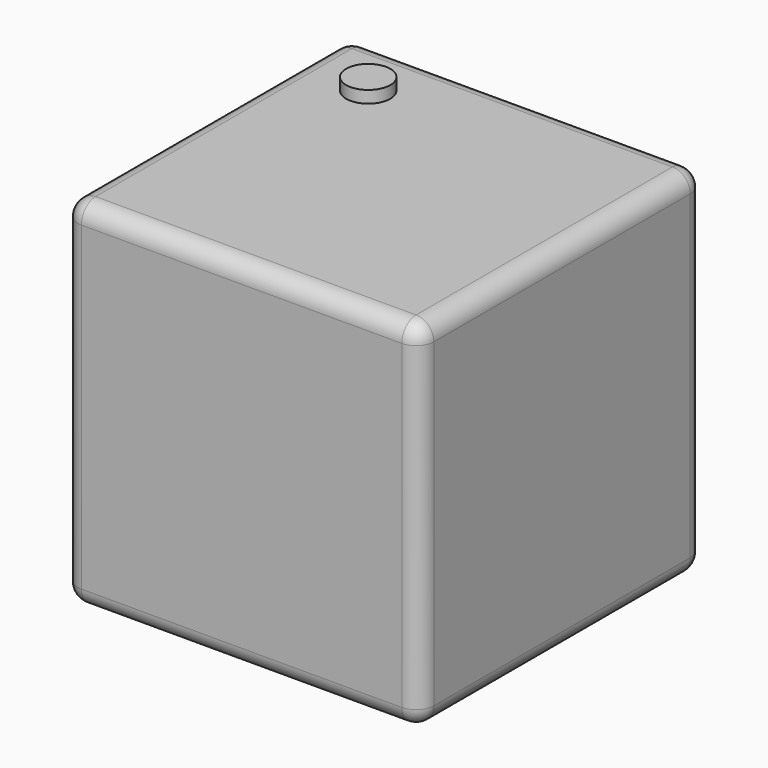
from build123d import *

# Parameters (mm, degrees)
F0_W         = 100
F0_H         = 100
F1_DEPTH     = 100
F2_R         = 5
F3_W         = 84.485553205
F3_H         = 83.5751444101
F4_DEPTH     = 96.9
F5_R         = 5
F6_T1_DEPTH  = 84.485553205
F6_T3_DEPTH  = 83.5751444101
F6_T9_DEPTH  = 96.985553205
F6_T13_DEPTH = 96.0751444101
F6_T20_DEPTH = 96.985553205
F6_T24_DEPTH = 96.0751444101
F6_T31_DEPTH = 96.0751444101
F6_T35_DEPTH = 96.985553205
F6_T42_DEPTH = 96.0751444101
F6_T46_DEPTH = 96.985553205
F7_R         = 6.1934205271
F8_DEPTH     = 3.4


# Not quite as in the source:
# - a fillet or chamfer that OpenCascade refuses, or shapes differently, is made with other operations: its cross-section is extruded or revolved along the edge and cut away or added


with BuildPart() as f1:
    # F0 (on Front) → F1 (new body)
    with BuildSketch(Plane.XZ):
        Rectangle(F0_W, F0_H)
    extrude(amount=F1_DEPTH)

    # F2
    f2_edges = [f1.edges().sort_by_distance(p)[0] for p in [
        (0, -100, 50),
        (-50, -100, 0),
        (0, -100, -50),
        (50, -100, 0),
        (50, -50, -50),
        (-50, -50, -50),
        (0, 0, -50),
        (50, -50, 50),
        (-50, -50, 50),
        (0, 0, 50),
        (50, 0, 0),
        (-50, 0, 0),
    ]]
    fillet(f2_edges, radius=F2_R)

    # F3 (on Front) → F4 (cut)
    with BuildSketch(Plane.XZ):
        Rectangle(F3_W, F3_H)
    extrude(amount=F4_DEPTH, mode=Mode.SUBTRACT)

    # F5
    f5_edges = [f1.edges().sort_by_distance(p)[0] for p in [
        (0, -96.9, -41.787572),
        (42.242777, -96.9, 0),
        (0, -96.9, 41.787572),
        (-42.242777, -96.9, 0),
    ]]
    fillet(f5_edges, radius=F5_R)

    # F6: fillet of radius 5 on 8 edges, made by hand

    # F6_s2 → F6_t1 (cut)
    with BuildSketch(Plane.YZ.offset(-42.2427766025)):
        with BuildLine():
            ThreePointArc((-5, -41.7875722051), (-1.4644660941, -43.2520382991), (0, -46.7875722051))
            Line((0, -46.7875722051), (0, -41.7875722051))
            Line((0, -41.7875722051), (-5, -41.7875722051))
        make_face()
        with BuildLine():
            ThreePointArc((0, 46.7875722051), (-1.4644660941, 43.2520382991), (-5, 41.7875722051))
            Line((-5, 41.7875722051), (0, 41.7875722051))
            Line((0, 41.7875722051), (0, 46.7875722051))
        make_face()
    extrude(amount=F6_T1_DEPTH, mode=Mode.SUBTRACT)

    # F6_s4 → F6_t3 (cut)
    with BuildSketch(Plane.XY.offset(-41.7875722051)):
        with BuildLine():
            ThreePointArc((47.2427766025, 0), (43.7072426966, -1.4644660941), (42.2427766025, -5))
            Line((42.2427766025, -5), (42.2427766025, 0))
            Line((42.2427766025, 0), (47.2427766025, 0))
        make_face()
        with BuildLine():
            ThreePointArc((-42.2427766025, -5), (-43.7072426966, -1.4644660941), (-47.2427766025, 0))
            Line((-47.2427766025, 0), (-42.2427766025, 0))
            Line((-42.2427766025, 0), (-42.2427766025, -5))
        make_face()
    extrude(amount=F6_T3_DEPTH, mode=Mode.SUBTRACT)


with BuildPart() as f6_tool7:
    # F6_s8 → F6_t9 (new body)
    with BuildSketch(Plane.YZ.offset(-54.7427766025)):
        with BuildLine():
            ThreePointArc((-5, -41.7875722051), (-1.4644660941, -43.2520382991), (0, -46.7875722051))
            Line((0, -46.7875722051), (0, -41.7875722051))
            Line((0, -41.7875722051), (-5, -41.7875722051))
        make_face()
    extrude(amount=F6_T9_DEPTH)

    split(bisect_by=Plane.YZ.offset(-42.2427766025), keep=Keep.BOTTOM)


with BuildPart() as f6_tool11:
    # F6_s12 → F6_t13 (new body)
    with BuildSketch(Plane.XY.offset(41.7875722051)):
        with BuildLine():
            ThreePointArc((-42.2427766025, -5), (-43.7072426966, -1.4644660941), (-47.2427766025, 0))
            Line((-47.2427766025, 0), (-42.2427766025, 0))
            Line((-42.2427766025, 0), (-42.2427766025, -5))
        make_face()
    extrude(amount=-F6_T13_DEPTH)

    split(bisect_by=Plane.XY.offset(-41.7875722051), keep=Keep.BOTTOM)


with BuildPart() as f6_tool7_1:
    add(f6_tool7.part)

    # F6_t15: intersect F6_tool11
    add(f6_tool11.part, mode=Mode.INTERSECT)


with BuildPart() as f1_1:
    add(f1.part)

    # F6_t5: cut F6_tool7
    add(f6_tool7_1.part, mode=Mode.SUBTRACT)


with BuildPart() as f6_tool18:
    # F6_s19 → F6_t20 (new body)
    with BuildSketch(Plane.YZ.offset(-42.2427766025)):
        with BuildLine():
            ThreePointArc((-5, -41.7875722051), (-1.4644660941, -43.2520382991), (0, -46.7875722051))
            Line((0, -46.7875722051), (0, -41.7875722051))
            Line((0, -41.7875722051), (-5, -41.7875722051))
        make_face()
    extrude(amount=F6_T20_DEPTH)

    split(bisect_by=Plane.YZ.offset(42.2427766025), keep=Keep.TOP)


with BuildPart() as f6_tool22:
    # F6_s23 → F6_t24 (new body)
    with BuildSketch(Plane.XY.offset(-54.2875722051)):
        with BuildLine():
            ThreePointArc((47.2427766025, 0), (43.7072426966, -1.4644660941), (42.2427766025, -5))
            Line((42.2427766025, -5), (42.2427766025, 0))
            Line((42.2427766025, 0), (47.2427766025, 0))
        make_face()
    extrude(amount=F6_T24_DEPTH)

    split(bisect_by=Plane.XY.offset(-41.7875722051), keep=Keep.BOTTOM)


with BuildPart() as f6_tool18_1:
    add(f6_tool18.part)

    # F6_t26: intersect F6_tool22
    add(f6_tool22.part, mode=Mode.INTERSECT)


with BuildPart() as f1_2:
    add(f1_1.part)

    # F6_t16: cut F6_tool18
    add(f6_tool18_1.part, mode=Mode.SUBTRACT)


with BuildPart() as f6_tool29:
    # F6_s30 → F6_t31 (new body)
    with BuildSketch(Plane.XY.offset(-41.7875722051)):
        with BuildLine():
            ThreePointArc((47.2427766025, 0), (43.7072426966, -1.4644660941), (42.2427766025, -5))
            Line((42.2427766025, -5), (42.2427766025, 0))
            Line((42.2427766025, 0), (47.2427766025, 0))
        make_face()
    extrude(amount=F6_T31_DEPTH)

    split(bisect_by=Plane.XY.offset(41.7875722051), keep=Keep.TOP)


with BuildPart() as f6_tool33:
    # F6_s34 → F6_t35 (new body)
    with BuildSketch(Plane.YZ.offset(54.7427766025)):
        with BuildLine():
            ThreePointArc((0, 46.7875722051), (-1.4644660941, 43.2520382991), (-5, 41.7875722051))
            Line((-5, 41.7875722051), (0, 41.7875722051))
            Line((0, 41.7875722051), (0, 46.7875722051))
        make_face()
    extrude(amount=-F6_T35_DEPTH)

    split(bisect_by=Plane.YZ.offset(42.2427766025), keep=Keep.TOP)


with BuildPart() as f6_tool29_1:
    add(f6_tool29.part)

    # F6_t37: intersect F6_tool33
    add(f6_tool33.part, mode=Mode.INTERSECT)


with BuildPart() as f1_3:
    add(f1_2.part)

    # F6_t27: cut F6_tool29
    add(f6_tool29_1.part, mode=Mode.SUBTRACT)


with BuildPart() as f6_tool40:
    # F6_s41 → F6_t42 (new body)
    with BuildSketch(Plane.XY.offset(54.2875722051)):
        with BuildLine():
            ThreePointArc((-42.2427766025, -5), (-43.7072426966, -1.4644660941), (-47.2427766025, 0))
            Line((-47.2427766025, 0), (-42.2427766025, 0))
            Line((-42.2427766025, 0), (-42.2427766025, -5))
        make_face()
    extrude(amount=-F6_T42_DEPTH)

    split(bisect_by=Plane.XY.offset(41.7875722051), keep=Keep.TOP)


with BuildPart() as f6_tool44:
    # F6_s45 → F6_t46 (new body)
    with BuildSketch(Plane.YZ.offset(42.2427766025)):
        with BuildLine():
            ThreePointArc((0, 46.7875722051), (-1.4644660941, 43.2520382991), (-5, 41.7875722051))
            Line((-5, 41.7875722051), (0, 41.7875722051))
            Line((0, 41.7875722051), (0, 46.7875722051))
        make_face()
    extrude(amount=-F6_T46_DEPTH)

    split(bisect_by=Plane.YZ.offset(-42.2427766025), keep=Keep.BOTTOM)


with BuildPart() as f6_tool40_1:
    add(f6_tool40.part)

    # F6_t48: intersect F6_tool44
    add(f6_tool44.part, mode=Mode.INTERSECT)


with BuildPart() as f1_4:
    add(f1_3.part)

    # F6_t38: cut F6_tool40
    add(f6_tool40_1.part, mode=Mode.SUBTRACT)

    # F7 (on face) → F8 (join)
    with BuildSketch(Plane.XY.offset(50)):
        with Locations((-29.7398809344, -18.3617770672)):
            Circle(F7_R)
    extrude(amount=F8_DEPTH)


solid = f1_4.part
